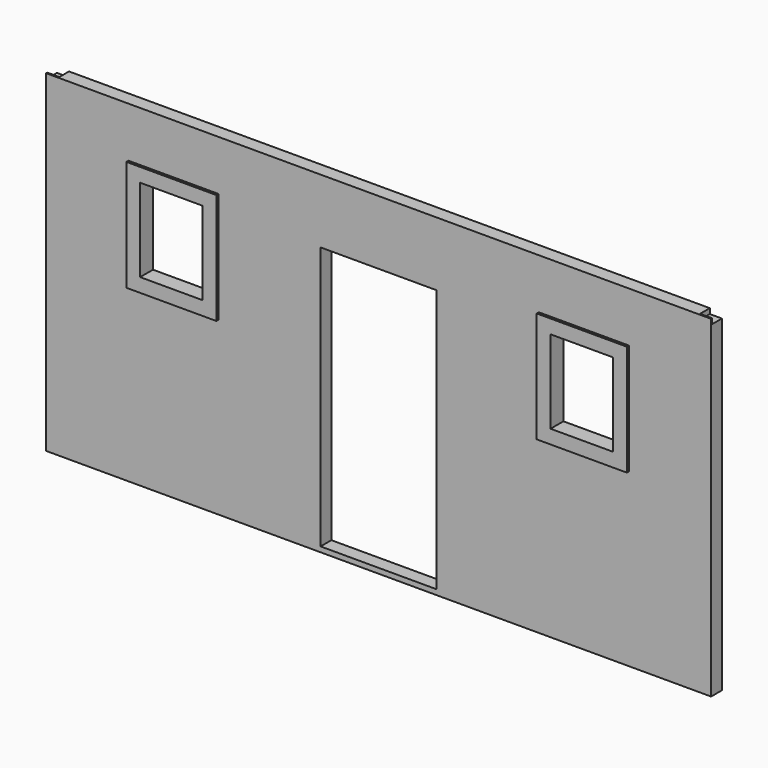
from build123d import *

# Parameters (mm, degrees)
F0_W     = 38.1
F0_H     = 2324.1
F0_H_2   = 609.6
F0_W_2   = 4699
F0_H_3   = 38.1
F0_H_4   = 1930.4
F0_H_5   = 1282.7
F1_DEPTH = 88.9
F2_W     = 850.9
F2_H     = 1930.4
F2_W_2   = 457.2
F2_H_2   = 609.6
F3_DEPTH = 10.16
F4_W     = 660.4
F4_H     = 812.8
F4_W_2   = 457.2
F4_H_2   = 609.6
F5_DEPTH = 19.05


# Not quite as in the source:
# - a feature names something its author has since deleted; it is built from what else it names


with BuildPart() as f1:
    # F0 (on Front) → F1 (new body)
    with BuildSketch(Plane.XZ):
        with Locations((19.05, 1200.15)):
            Rectangle(F0_W, F0_H)
        with Locations((57.15, 1200.15)):
            Rectangle(F0_W, F0_H)
        Polygon((0, 38.1), (0, 0), (4876.8, 0), (4876.8, 38.1), (4838.7, 38.1), (4800.6, 38.1), (4540.25, 38.1), (4502.15, 38.1), (4248.15, 38.1), (4210.05, 38.1), (4171.95, 38.1), (3714.75, 38.1), (3676.65, 38.1), (3638.55, 38.1), (3308.35, 38.1), (3270.25, 38.1), (2940.05, 38.1), (2901.95, 38.1), (2863.85, 38.1), (2012.95, 38.1), (1974.85, 38.1), (1936.75, 38.1), (1606.55, 38.1), (1568.45, 38.1), (1238.25, 38.1), (1200.15, 38.1), (1162.05, 38.1), (704.85, 38.1), (666.75, 38.1), (628.65, 38.1), (374.65, 38.1), (336.55, 38.1), (76.2, 38.1), (38.1, 38.1), align=None)
        with Locations((355.6, 1200.15)):
            Rectangle(F0_W, F0_H)
        Polygon((628.65, 2362.2), (628.65, 38.1), (666.75, 38.1), (666.75, 1320.8), (666.75, 1358.9), (666.75, 1968.5), (666.75, 2057.4), (666.75, 2362.2), align=None)
        Polygon((1200.15, 1320.8), (1200.15, 38.1), (1238.25, 38.1), (1238.25, 2362.2), (1200.15, 2362.2), (1200.15, 2057.4), (1200.15, 1968.5), (1200.15, 1358.9), align=None)
        Polygon((895.35, 2057.4), (666.75, 2057.4), (666.75, 1968.5), (704.85, 1968.5), (1162.05, 1968.5), (1200.15, 1968.5), (1200.15, 2057.4), (933.45, 2057.4), align=None)
        with Locations((685.8, 1663.7)):
            Rectangle(F0_W, F0_H_2)
        with Locations((1181.1, 1663.7)):
            Rectangle(F0_W, F0_H_2)
        Polygon((666.75, 1358.9), (666.75, 1320.8), (704.85, 1320.8), (1162.05, 1320.8), (1200.15, 1320.8), (1200.15, 1358.9), (1162.05, 1358.9), (704.85, 1358.9), align=None)
        Polygon((0, 2400.3), (0, 2362.2), (38.1, 2362.2), (76.2, 2362.2), (336.55, 2362.2), (374.65, 2362.2), (628.65, 2362.2), (666.75, 2362.2), (895.35, 2362.2), (933.45, 2362.2), (1200.15, 2362.2), (1238.25, 2362.2), (1568.45, 2362.2), (1606.55, 2362.2), (1936.75, 2362.2), (1974.85, 2362.2), (2901.95, 2362.2), (2940.05, 2362.2), (3270.25, 2362.2), (3308.35, 2362.2), (3638.55, 2362.2), (3676.65, 2362.2), (4210.05, 2362.2), (4248.15, 2362.2), (4502.15, 2362.2), (4540.25, 2362.2), (4800.6, 2362.2), (4838.7, 2362.2), (4876.8, 2362.2), (4876.8, 2400.3), (4787.9, 2400.3), (88.9, 2400.3), align=None)
        with Locations((2438.4, 2419.35)):
            Rectangle(F0_W_2, F0_H_3)
        with Locations((1587.5, 1200.15)):
            Rectangle(F0_W, F0_H)
        with Locations((4857.75, 1200.15)):
            Rectangle(F0_W, F0_H)
        with Locations((4819.65, 1200.15)):
            Rectangle(F0_W, F0_H)
        with Locations((3289.3, 1200.15)):
            Rectangle(F0_W, F0_H)
        Polygon((4171.95, 1320.8), (4210.05, 1320.8), (4210.05, 1358.9), (4171.95, 1358.9), (3714.75, 1358.9), (3676.65, 1358.9), (3676.65, 1320.8), (3714.75, 1320.8), align=None)
        with Locations((3695.7, 1663.7)):
            Rectangle(F0_W, F0_H_2)
        Polygon((3676.65, 2057.4), (3676.65, 2362.2), (3638.55, 2362.2), (3638.55, 38.1), (3676.65, 38.1), (3676.65, 1320.8), (3676.65, 1358.9), (3676.65, 1968.5), align=None)
        with Locations((4191, 1663.7)):
            Rectangle(F0_W, F0_H_2)
        Polygon((4210.05, 38.1), (4248.15, 38.1), (4248.15, 2362.2), (4210.05, 2362.2), (4210.05, 2057.4), (4210.05, 1968.5), (4210.05, 1358.9), (4210.05, 1320.8), align=None)
        Polygon((4210.05, 1968.5), (4210.05, 2057.4), (3676.65, 2057.4), (3676.65, 1968.5), (3714.75, 1968.5), (4171.95, 1968.5), align=None)
        with Locations((4521.2, 1200.15)):
            Rectangle(F0_W, F0_H)
        Polygon((1936.75, 2362.2), (1936.75, 38.1), (1974.85, 38.1), (1974.85, 1968.5), (1974.85, 2057.4), (1974.85, 2362.2), align=None)
        Polygon((2940.05, 38.1), (2940.05, 2362.2), (2901.95, 2362.2), (2901.95, 2057.4), (2901.95, 1968.5), (2901.95, 38.1), align=None)
        with Locations((1993.9, 1003.3)):
            Rectangle(F0_W, F0_H_4)
        Polygon((2901.95, 1968.5), (2901.95, 2057.4), (1974.85, 2057.4), (1974.85, 1968.5), (2012.95, 1968.5), (2863.85, 1968.5), align=None)
        with Locations((2882.9, 1003.3)):
            Rectangle(F0_W, F0_H_4)
        with Locations((3695.7, 679.45)):
            Rectangle(F0_W, F0_H_5)
        with Locations((4191, 679.45)):
            Rectangle(F0_W, F0_H_5)
        with Locations((685.8, 679.45)):
            Rectangle(F0_W, F0_H_5)
        with Locations((1181.1, 679.45)):
            Rectangle(F0_W, F0_H_5)
    extrude(amount=F1_DEPTH)

    # F2 (on face) → F3 (join)
    with BuildSketch(Plane.XZ.offset(88.9)):
        Polygon((0, 2400.3), (0, 0), (4876.8, 0), (4876.8, 2400.3), (4876.8, 2438.4), (4787.9, 2438.4), (88.9, 2438.4), (0, 2438.4), align=None)
        with Locations((2438.4, 1003.3)):
            Rectangle(F2_W, F2_H, mode=Mode.SUBTRACT)
        with Locations((933.45, 1663.7)):
            Rectangle(F2_W_2, F2_H_2, mode=Mode.SUBTRACT)
        with Locations((3943.35, 1663.7)):
            Rectangle(F2_W_2, F2_H_2, mode=Mode.SUBTRACT)
    extrude(amount=F3_DEPTH)

    # F4 (on face) → F5 (join)
    with BuildSketch(Plane.XZ.offset(99.06)):
        with Locations((933.45, 1663.7)):
            Rectangle(F4_W, F4_H)
        with Locations((933.45, 1663.7)):
            Rectangle(F4_W_2, F4_H_2, mode=Mode.SUBTRACT)
        with Locations((3943.35, 1663.7)):
            Rectangle(F4_W, F4_H)
        with Locations((3943.35, 1663.7)):
            Rectangle(F4_W_2, F4_H_2, mode=Mode.SUBTRACT)
    extrude(amount=F5_DEPTH)


solid = f1.part
